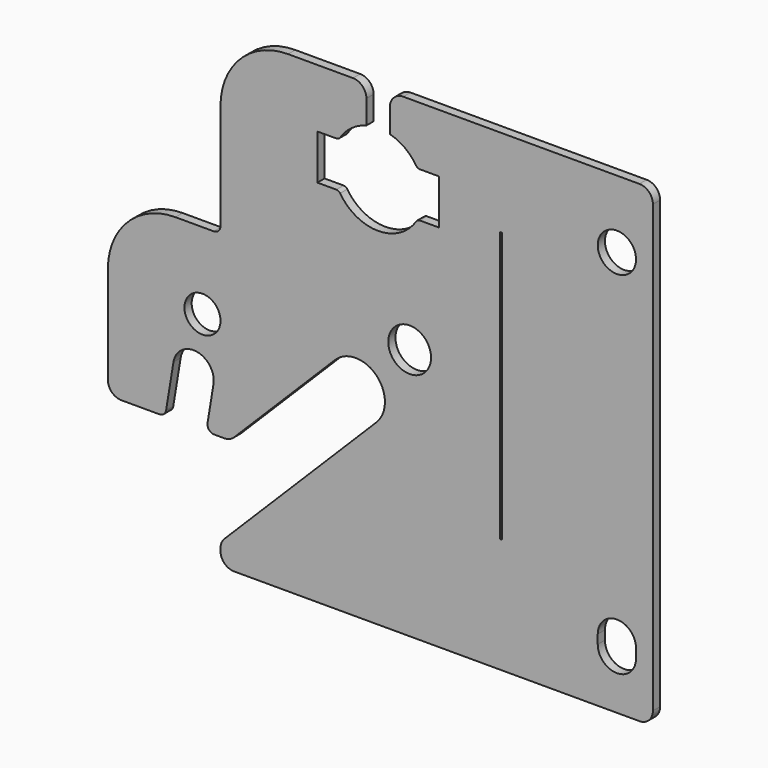
from build123d import *

# Parameters (mm, degrees)
F0_R     = 4
F0_R_2   = 4.75
F0_W     = 0.5
F0_H     = 60
F0_R_3   = 4.25
F1_DEPTH = 2
F2_R     = 15
F3_R     = 3
F4_R     = 1.5
F5_R     = 1


# Not quite as in the source:
# - a feature names something its author has since deleted; it is built from what else it names


with BuildPart() as f1:
    # F0 (on Front) → F1 (new body)
    with BuildSketch(Plane.XZ):
        with BuildLine():
            Line((159.6967741251, 4.7991039181), (159.6967741251, 0))
            Line((159.6967741251, 0), (255.6967741251, 0))
            Line((255.6967741251, 0), (255.6967741251, 105))
            Line((255.6967741251, 105), (197.2967741251, 105))
            Line((197.2967741251, 105), (197.2967741251, 96.7078576421))
            ThreePointArc((197.2967741251, 96.7078576421), (200.8257976645, 94.9647705839), (203.4147153958, 92))
            Line((203.4147153958, 92), (208.1967741251, 92))
            Line((208.1967741251, 92), (208.1967741251, 82))
            Line((208.1967741251, 82), (203.4147153958, 82))
            ThreePointArc((203.4147153958, 82), (194.6967741251, 76.95), (185.9788328544, 82))
            Line((185.9788328544, 82), (181.1967741251, 82))
            Line((181.1967741251, 82), (181.1967741251, 92))
            Line((181.1967741251, 92), (185.9788328544, 92))
            ThreePointArc((185.9788328544, 92), (188.5677505857, 94.9647705839), (192.0967741251, 96.7078576421))
            Line((192.0967741251, 96.7078576421), (192.0967741251, 105))
            Line((192.0967741251, 105), (159.6967741251, 105))
            Line((159.6967741251, 105), (159.6967741251, 65))
            Line((159.6967741251, 65), (134.6967741251, 65))
            Line((134.6967741251, 65), (134.6967741251, 25.3155251003))
            Line((134.6967741251, 25.3155251003), (147.4130505224, 25.3155251003))
            Line((147.4130505224, 25.3155251003), (149.2561978018, 36.5444159815))
            ThreePointArc((149.2561978018, 36.5444159815), (154.4256650063, 40.2561014236), (158.1373504484, 35.0866342191))
            Line((158.1373504484, 35.0866342191), (156.5334882879, 25.3155251003))
            Line((156.5334882879, 25.3155251003), (161.81991107, 25.3155251003))
            Line((161.81991107, 25.3155251003), (163.0631786775, 26.5587927078))
            Line((163.0631786775, 26.5587927078), (184.9027867776, 48.3984008079))
            ThreePointArc((184.9027867776, 48.3984008079), (194.1972390474, 48.6983039321), (194.2972221661, 39.399551959))
            Line((194.2972221661, 39.399551959), (159.6967741251, 4.7991039181))
        make_face()
        with Locations((155.6967741251, 48)):
            Circle(F0_R, mode=Mode.SUBTRACT)
        with BuildLine():
            ThreePointArc((251.9467741251, 12), (247.6967741251, 7.75), (243.4467741251, 12))
            Line((243.4467741251, 12), (243.4467741251, 14))
            ThreePointArc((243.4467741251, 14), (247.6967741251, 18.25), (251.9467741251, 14))
            Line((251.9467741251, 14), (251.9467741251, 12))
        make_face(mode=Mode.SUBTRACT)
        with Locations((201.6967741251, 56)):
            Circle(F0_R_2, mode=Mode.SUBTRACT)
        with Locations((221.9467741251, 55.5368482322)):
            Rectangle(F0_W, F0_H, mode=Mode.SUBTRACT)
        with Locations((247.6967741251, 90)):
            Circle(F0_R_3, mode=Mode.SUBTRACT)
    extrude(amount=F1_DEPTH)

    # F2
    f2_edges = [f1.edges().sort_by_distance(p)[0] for p in [
        (134.696774, -1, 65),
        (159.696774, -1, 105),
    ]]
    fillet(f2_edges, radius=F2_R)

    # F3
    f3_edges = [f1.edges().sort_by_distance(p)[0] for p in [
        (255.696774, -1, 105),
        (255.696774, -1, 0),
        (197.296774, -1, 105),
        (192.096774, -1, 105),
        (161.819911, -1, 25.315525),
        (159.696774, -1, 4.799104),
        (159.696774, -1, 0),
        (134.696774, -1, 25.315525),
    ]]
    fillet(f3_edges, radius=F3_R)

    # F4
    f4_edges = [f1.edges().sort_by_distance(p)[0] for p in [
        (147.413051, -1, 25.315525),
        (156.533488, -1, 25.315525),
        (159.696774, -1, 65),
    ]]
    fillet(f4_edges, radius=F4_R)

    # F5
    f5_edges = [f1.edges().sort_by_distance(p)[0] for p in [
        (185.978833, -1, 92),
        (185.978833, -1, 82),
        (203.414715, -1, 92),
        (203.414715, -1, 82),
    ]]
    fillet(f5_edges, radius=F5_R)


solid = f1.part
